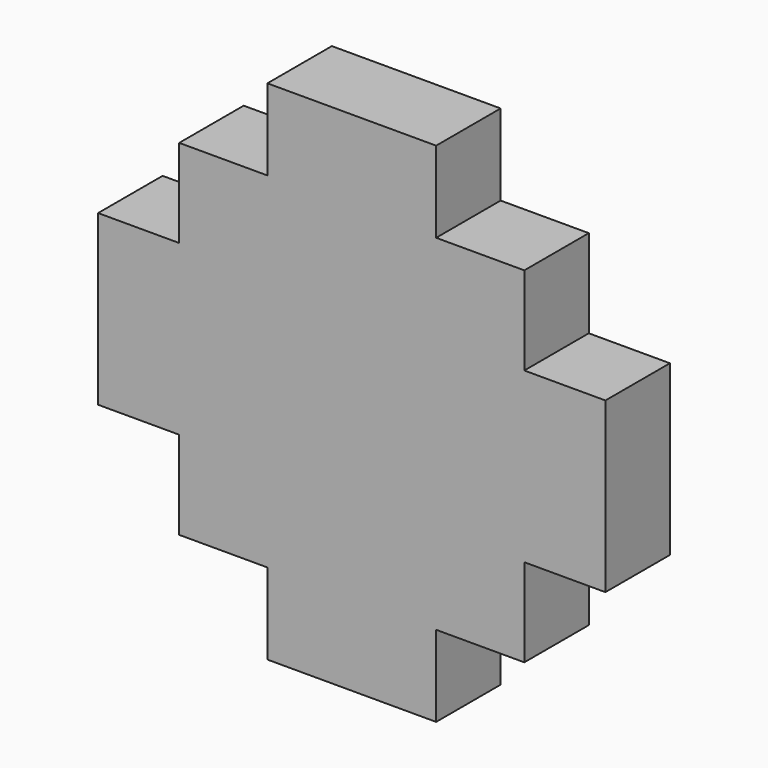
from build123d import *

# Parameters (mm, degrees)
F1_DEPTH     = 2.032
F3_TEXT_SIZE = 8.5776133364
F4_DEPTH     = 0.508


# Not quite as in the source:
# - Text() gives the source's letters only with a copy of the font that has no kerning and outlines rounded to 1/6400 em; it was checked with that copy


with BuildPart() as f1:
    # F0 (on Front) → F1 (new body)
    with BuildSketch(Plane.XZ):
        Polygon((-15.2212520439, 36.2265945869), (-17.3485020439, 36.2265945869), (-19.4757520439, 36.2265945869), (-19.4757520439, 34.1818945869), (-21.6982520439, 34.1818945869), (-21.6982520439, 31.9593945869), (-23.7429520439, 31.9593945869), (-23.7429520439, 29.8321445869), (-23.7429520439, 27.7048945869), (-21.6982520439, 27.7048945869), (-21.6982520439, 25.4823945869), (-19.4757520439, 25.4823945869), (-19.4757520439, 23.4376945869), (-17.3485020439, 23.4376945869), (-15.2212520439, 23.4376945869), (-15.2212520439, 25.4823945869), (-12.9987520439, 25.4823945869), (-12.9987520439, 27.7048945869), (-10.9540520439, 27.7048945869), (-10.9540520439, 29.8321445869), (-10.9540520439, 31.9593945869), (-12.9987520439, 31.9593945869), (-12.9987520439, 34.1818945869), (-15.2212520439, 34.1818945869), align=None)
    extrude(amount=F1_DEPTH)

    # F3 (on offset) → F4 (cut)
    with BuildSketch(Plane.XZ.offset(4.064)):
        with Locations((-20.2790203011, 26.6853499193)):
            Text('K', F3_TEXT_SIZE, font='Open Sans', text_align=(TextAlign.LEFT, TextAlign.BOTTOM))
    extrude(amount=-F4_DEPTH, mode=Mode.SUBTRACT)


solid = f1.part
